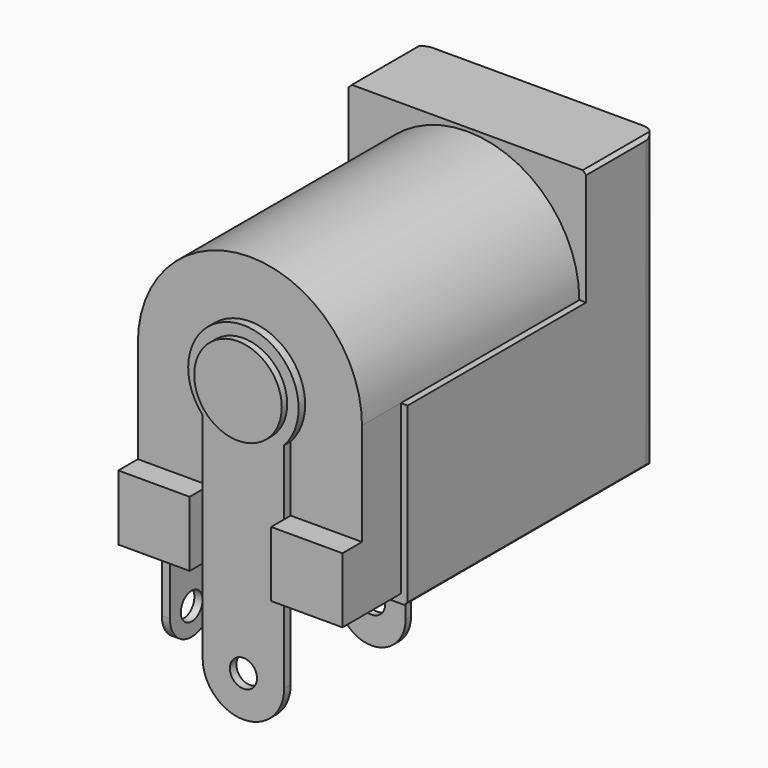
from build123d import *

# Parameters (mm, degrees)
F0_W      = 8.89
F0_H      = 10.922
F1_DEPTH  = 3.302
F3_DEPTH  = 13.462
F4_R      = 0.508
F4_R_2    = 1.6374420612
F5_DEPTH  = 0.3048
F6_R      = 1.6374420612
F7_DEPTH  = 0.254
F8_W      = 8.89
F8_H      = 6.604
F9_DEPTH  = 8.3439
F10_W     = 2.667
F10_H     = 2.4411697693
F11_DEPTH = 0.3048
F12_W     = 2.667
F12_H     = 2.4411697693
F13_DEPTH = 0.6096
F14_R     = 2.75
F15_DEPTH = 5.08
F16_SIZE  = 0.127
F18_R     = 0.508
F19_DEPTH = 0.254
F20_R     = 0.508
F21_DEPTH = 0.3048
F22_R     = 0.254
F23_R     = 1.016
F24_DEPTH = 4.5974
F25_R     = 1.016
F26_R     = 0.508


with BuildPart() as f1:
    # F0 (on Front) → F1 (new body)
    with BuildSketch(Plane.XZ):
        with Locations((0, -1.143)):
            Rectangle(F0_W, F0_H)
    extrude(amount=F1_DEPTH)

    # F2 (on face) → F3 (join)
    with BuildSketch(Plane(origin=(0, 0, 0), x_dir=(-1, 0, 0), z_dir=(0, 1, 0))):
        with BuildLine():
            ThreePointArc((4.191, 0), (0, 4.191), (-4.191, 0))
            Line((-4.191, 0), (-4.191, -6.2759071589))
            Line((-4.191, -6.2759071589), (4.191, -6.2759071589))
            Line((4.191, -6.2759071589), (4.191, 0))
        make_face()
    extrude(amount=-F3_DEPTH)

    # F4 (on face) → F5 (join)
    with BuildSketch(Plane.XZ.offset(13.462)):
        with BuildLine():
            Line((1.524, -9.398), (1.524, -1.3935676202))
            ThreePointArc((1.524, -1.3935676202), (0, 2.0650924222), (-1.524, -1.3935676202))
            Line((-1.524, -1.3935676202), (-1.524, -9.398))
            ThreePointArc((-1.524, -9.398), (-1.0776307345, -10.4756307345), (0, -10.922))
            ThreePointArc((0, -10.922), (1.0776307345, -10.4756307345), (1.524, -9.398))
        make_face()
        with Locations((0, -9.398)):
            Circle(F4_R, mode=Mode.SUBTRACT)
        Circle(F4_R_2, mode=Mode.SUBTRACT)
        Circle(F4_R_2)
    extrude(amount=F5_DEPTH)

    # F6 (on face) → F7 (join)
    with BuildSketch(Plane.XZ.offset(13.7668)):
        Circle(F6_R)
    extrude(amount=F7_DEPTH)

    # F8 (on face) → F9 (join)
    with BuildSketch(Plane.XZ.offset(3.302)):
        with Locations((0, -3.302)):
            Rectangle(F8_W, F8_H)
    extrude(amount=F9_DEPTH)

    # F10 (on face) → F11 (join, through all)
    with BuildSketch(Plane.XZ.offset(13.462)):
        with Locations((-2.8575, -5.0553222742)):
            Rectangle(F10_W, F10_H)
        with Locations((2.8575, -5.0553222742)):
            Rectangle(F10_W, F10_H)
    extrude(amount=F11_DEPTH)

    # F12 (on face) → F13 (join)
    with BuildSketch(Plane.XZ.offset(13.7668)):
        with Locations((-2.8575, -5.0553222742)):
            Rectangle(F12_W, F12_H)
        with Locations((2.8575, -5.0553222742)):
            Rectangle(F12_W, F12_H)
    extrude(amount=F13_DEPTH)

    # F14 (on face) → F15 (cut)
    with BuildSketch(Plane(origin=(0, 0, 0), x_dir=(-1, 0, 0), z_dir=(0, 1, 0))):
        Circle(F14_R)
    extrude(amount=-F15_DEPTH, mode=Mode.SUBTRACT)

    # F16
    f16_edges = [f1.edges().sort_by_distance(p)[0] for p in [
        (-4.445, -1.651, 4.318),
        (4.445, -1.651, 4.318),
        (4.445, -5.82295, -6.604),
        (-4.445, -5.82295, -6.604),
        (2.75, 0, 0),
    ]]
    chamfer(f16_edges, length=F16_SIZE)

    # F18 (on offset) → F19 (join)
    with BuildSketch(Plane.XZ.offset(7.7724)):
        with BuildLine():
            Line((1.27, -6.604), (-1.27, -6.604))
            Line((-1.27, -6.604), (-1.27, -9.652))
            ThreePointArc((-1.27, -9.652), (-0.8980256121, -10.5500256121), (0, -10.922))
            ThreePointArc((0, -10.922), (0.8980256121, -10.5500256121), (1.27, -9.652))
            Line((1.27, -9.652), (1.27, -6.604))
        make_face()
        with Locations((0, -9.398)):
            Circle(F18_R, mode=Mode.SUBTRACT)
    extrude(amount=-F19_DEPTH)

    # F20 (on face) → F21 (join)
    with BuildSketch(Plane(origin=(-4.445, 0, 0), x_dir=(0, -1, 0), z_dir=(-1, 0, 0))):
        with BuildLine():
            Line((11.6459, -3.0857360969), (9.6139, -3.0857360969))
            Line((9.6139, -3.0857360969), (9.6139, -9.906))
            ThreePointArc((9.6139, -9.906), (9.9114795103, -10.6244204897), (10.6299, -10.922))
            ThreePointArc((10.6299, -10.922), (11.3483204897, -10.6244204897), (11.6459, -9.906))
            Line((11.6459, -9.906), (11.6459, -3.0857360969))
        make_face()
        with Locations((10.6299, -9.906)):
            Circle(F20_R, mode=Mode.SUBTRACT)
    extrude(amount=F21_DEPTH)

    # F22
    f22_edges = [f1.edges().sort_by_distance(p)[0] for p in [
        (-4.7498, -10.6299, -3.085736),
    ]]
    fillet(f22_edges, radius=F22_R)

    # F23 (on face) → F24 (join)
    with BuildSketch(Plane(origin=(0, -5.08, 0), x_dir=(-1, 0, 0), z_dir=(0, 1, 0))):
        Circle(F23_R)
    extrude(amount=F24_DEPTH)

    # F25
    f25_edges = [f1.edges().sort_by_distance(p)[0] for p in [
        (1.016, -0.4826, 0),
    ]]
    fillet(f25_edges, radius=F25_R)

    # F26
    f26_edges = [f1.edges().sort_by_distance(p)[0] for p in [
        (-4.445, 0, -1.143),
        (4.445, 0, -1.143),
    ]]
    fillet(f26_edges, radius=F26_R)


solid = f1.part
